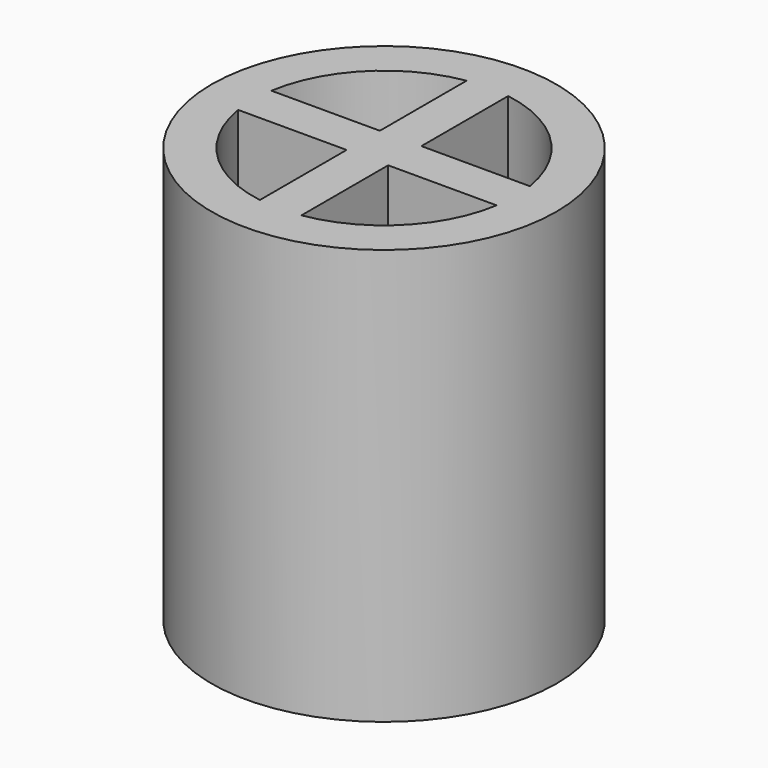
from build123d import *

# Parameters (mm, degrees)
F0_R     = 10.541
F1_DEPTH = 25.4
F2_R     = 8.001
F3_DEPTH = 22.86
F4_W     = 2.54
F4_H     = 2.54
F5_DEPTH = 22.86


with BuildPart() as f1:
    # F0 (on Top) → F1 (new body)
    with BuildSketch(Plane.XY):
        Circle(F0_R)
    extrude(amount=F1_DEPTH)

    # F2 (on face) → F3 (cut)
    with BuildSketch(Plane.XY.offset(25.4)):
        Circle(F2_R)
    extrude(amount=-F3_DEPTH, mode=Mode.SUBTRACT)

    # F4 (on face) → F5 (join)
    with BuildSketch(Plane.XY.offset(2.54)):
        Rectangle(F4_W, F4_H)
        with BuildLine():
            Line((1.27, 1.27), (1.27, -1.27))
            Line((1.27, -1.27), (7.8995633424, -1.27))
            ThreePointArc((7.8995633424, -1.27), (7.9756005198, -0.6370222515), (8.001, 0))
            ThreePointArc((8.001, 0), (7.9756005198, 0.6370222515), (7.8995633424, 1.27))
            Line((7.8995633424, 1.27), (1.27, 1.27))
        make_face()
        with BuildLine():
            Line((-1.27, -1.27), (-1.27, -7.8995633424))
            ThreePointArc((-1.27, -7.8995633424), (0, -8.001), (1.27, -7.8995633424))
            Line((1.27, -7.8995633424), (1.27, -1.27))
            Line((1.27, -1.27), (-1.27, -1.27))
        make_face()
        with BuildLine():
            Line((-7.8995633424, -1.27), (-1.27, -1.27))
            Line((-1.27, -1.27), (-1.27, 1.27))
            Line((-1.27, 1.27), (-7.8995633424, 1.27))
            ThreePointArc((-7.8995633424, 1.27), (-8.001, 0), (-7.8995633424, -1.27))
        make_face()
        with BuildLine():
            Line((-1.27, 7.8995633424), (-1.27, 1.27))
            Line((-1.27, 1.27), (1.27, 1.27))
            Line((1.27, 1.27), (1.27, 7.8995633424))
            ThreePointArc((1.27, 7.8995633424), (0, 8.001), (-1.27, 7.8995633424))
        make_face()
    extrude(amount=F5_DEPTH)


solid = f1.part
